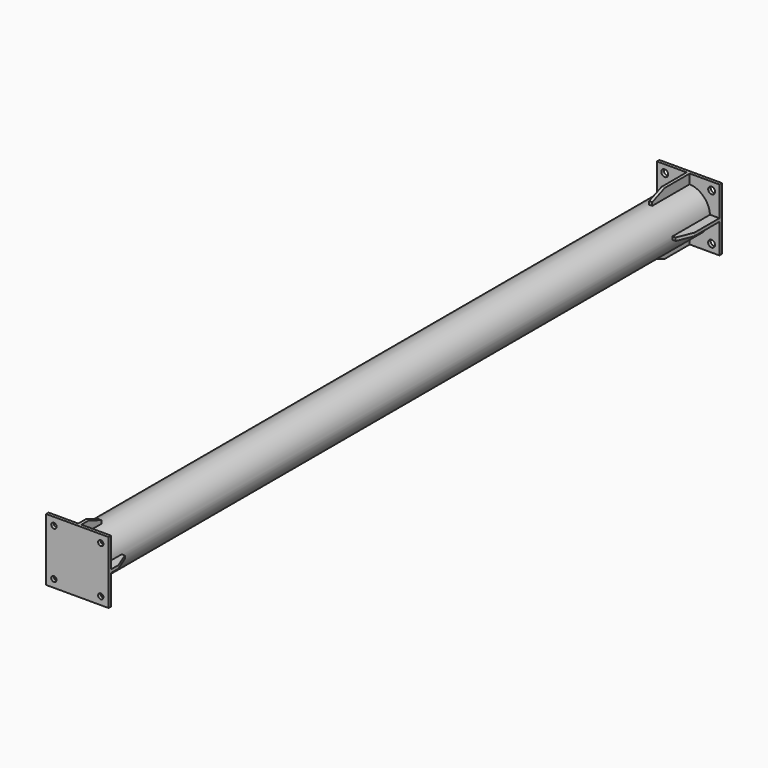
from build123d import *

# Parameters (mm, degrees)
F0_R          = 70
F0_R_2        = 65
F1_DEPTH      = 2434
F2_W          = 200
F2_H          = 200
F2_R          = 11
F3_DEPTH      = 10
F4_W          = 30.1787997812
F4_H          = 10
F4_W_2        = 10
F4_H_2        = 30.1787997812
F5_DEPTH      = 150
F6_T1_DEPTH   = 269.311363913
F6_T3_DEPTH   = 269.311363913
F6_T8_DEPTH   = 269.311363913
F6_S9_R       = 70
F6_T10_DEPTH  = 139
F8_W          = 200
F8_H          = 200
F8_R          = 8.5
F9_DEPTH      = 10
F10_W         = 10
F10_H         = 30.1787997812
F10_W_2       = 30.1787997812
F10_H_2       = 10
F11_DEPTH     = 80
F12_T1_DEPTH  = 269.311363913
F12_T3_DEPTH  = 269.311363913
F12_T8_DEPTH  = 269.311363913
F12_S9_R      = 70
F12_T10_DEPTH = 139
F12_T14_DEPTH = 269.311363913
F12_S15_R     = 70
F12_T16_DEPTH = 139


# Not quite as in the source:
# - a fillet or chamfer that OpenCascade refuses, or shapes differently, is made with other operations: its cross-section is extruded or revolved along the edge and cut away or added


with BuildPart() as f1:
    # F0 (on Front) → F1 (new body)
    with BuildSketch(Plane.XZ):
        Circle(F0_R)
        Circle(F0_R_2, mode=Mode.SUBTRACT)
    extrude(amount=F1_DEPTH)

    # F2 (on Front) → F3 (join)
    with BuildSketch(Plane.XZ):
        Rectangle(F2_W, F2_H)
        with Locations((-75, -75)):
            Circle(F2_R, mode=Mode.SUBTRACT)
        with Locations((75, -75)):
            Circle(F2_R, mode=Mode.SUBTRACT)
        with Locations((-75, 75)):
            Circle(F2_R, mode=Mode.SUBTRACT)
        with Locations((75, 75)):
            Circle(F2_R, mode=Mode.SUBTRACT)
    extrude(amount=-F3_DEPTH)

    # F4 (on Front) → F5 (join)
    with BuildSketch(Plane.XZ):
        with Locations((-84.9106001094, 0)):
            Rectangle(F4_W, F4_H)
        with Locations((0, 84.9106001094)):
            Rectangle(F4_W_2, F4_H_2)
        with Locations((84.9106001094, 0)):
            Rectangle(F4_W, F4_H)
        with Locations((0, -84.9106001094)):
            Rectangle(F4_W_2, F4_H_2)
    extrude(amount=F5_DEPTH)

    # F6: chamfer of 50 x 20 on 4 edges, made by hand

    # F6_s2 → F6_t1 (cut)
    with BuildSketch(Plane.YZ.offset(-134.6556819565)):
        Polygon((-100, 100), (-150, 80), (-150, 100), align=None)
        Polygon((-100, -100), (-150, -80), (-150, -100), align=None)
    extrude(amount=F6_T1_DEPTH, mode=Mode.SUBTRACT)

    # F6_s4 → F6_t3 (cut)
    with BuildSketch(Plane.XY.offset(-134.6556819565)):
        Polygon((100, -100), (80, -150), (100, -150), align=None)
    extrude(amount=F6_T3_DEPTH, mode=Mode.SUBTRACT)


with BuildPart() as f6_tool6:
    # F6_s7 → F6_t8 (new body)
    with BuildSketch(Plane.XY.offset(134.6556819565)):
        Polygon((-100, -130), (-50, -150), (-100, -150), align=None)
    extrude(amount=-F6_T8_DEPTH)

    # F6_s9 → F6_t10 (cut, symmetric)
    with BuildSketch(Plane.XZ.offset(140)):
        Circle(F6_S9_R)
    extrude(amount=F6_T10_DEPTH, both=True, mode=Mode.SUBTRACT)


with BuildPart() as f1_1:
    add(f1.part)

    # F6_t5: cut F6_tool6
    add(f6_tool6.part, mode=Mode.SUBTRACT)

    # F8 (on offset) → F9 (join)
    with BuildSketch(Plane.XZ.offset(2434)):
        Rectangle(F8_W, F8_H)
        with Locations((-75, -75)):
            Circle(F8_R, mode=Mode.SUBTRACT)
        with Locations((75, -75)):
            Circle(F8_R, mode=Mode.SUBTRACT)
        with Locations((-75, 75)):
            Circle(F8_R, mode=Mode.SUBTRACT)
        with Locations((75, 75)):
            Circle(F8_R, mode=Mode.SUBTRACT)
    extrude(amount=F9_DEPTH)

    # F10 (on face) → F11 (join)
    with BuildSketch(Plane(origin=(0, -2434, 0), x_dir=(-1, 0, 0), z_dir=(0, 1, 0))):
        with Locations((0, 84.9106001094)):
            Rectangle(F10_W, F10_H)
        with Locations((84.9106001094, 0)):
            Rectangle(F10_W_2, F10_H_2)
        with Locations((0, -84.9106001094)):
            Rectangle(F10_W, F10_H)
        with Locations((-84.9106001094, 0)):
            Rectangle(F10_W_2, F10_H_2)
    extrude(amount=F11_DEPTH)

    # F12: chamfer of 20 x 50 on 4 edges, made by hand

    # F12_s2 → F12_t1 (cut)
    with BuildSketch(Plane.YZ.offset(-134.6556819565)):
        Polygon((-2404, 100), (-2354, 80), (-2354, 100), align=None)
    extrude(amount=F12_T1_DEPTH, mode=Mode.SUBTRACT)

    # F12_s4 → F12_t3 (cut)
    with BuildSketch(Plane.XY.offset(-134.6556819565)):
        Polygon((100, -2404), (80, -2354), (100, -2354), align=None)
    extrude(amount=F12_T3_DEPTH, mode=Mode.SUBTRACT)


with BuildPart() as f12_tool6:
    # F12_s7 → F12_t8 (new body)
    with BuildSketch(Plane.XY.offset(-134.6556819565)):
        Polygon((-100, -2374), (-50, -2354), (-100, -2354), align=None)
    extrude(amount=F12_T8_DEPTH)

    # F12_s9 → F12_t10 (cut, symmetric)
    with BuildSketch(Plane.XZ.offset(2364)):
        Circle(F12_S9_R)
    extrude(amount=F12_T10_DEPTH, both=True, mode=Mode.SUBTRACT)


with BuildPart() as f1_2:
    add(f1_1.part)

    # F12_t5: cut F12_tool6
    add(f12_tool6.part, mode=Mode.SUBTRACT)


with BuildPart() as f12_tool12:
    # F12_s13 → F12_t14 (new body)
    with BuildSketch(Plane.YZ.offset(134.6556819565)):
        Polygon((-2374, -100), (-2354, -50), (-2354, -100), align=None)
    extrude(amount=-F12_T14_DEPTH)

    # F12_s15 → F12_t16 (cut, symmetric)
    with BuildSketch(Plane.XZ.offset(2364)):
        Circle(F12_S15_R)
    extrude(amount=F12_T16_DEPTH, both=True, mode=Mode.SUBTRACT)


with BuildPart() as f1_3:
    add(f1_2.part)

    # F12_t11: cut F12_tool12
    add(f12_tool12.part, mode=Mode.SUBTRACT)


solid = f1_3.part
